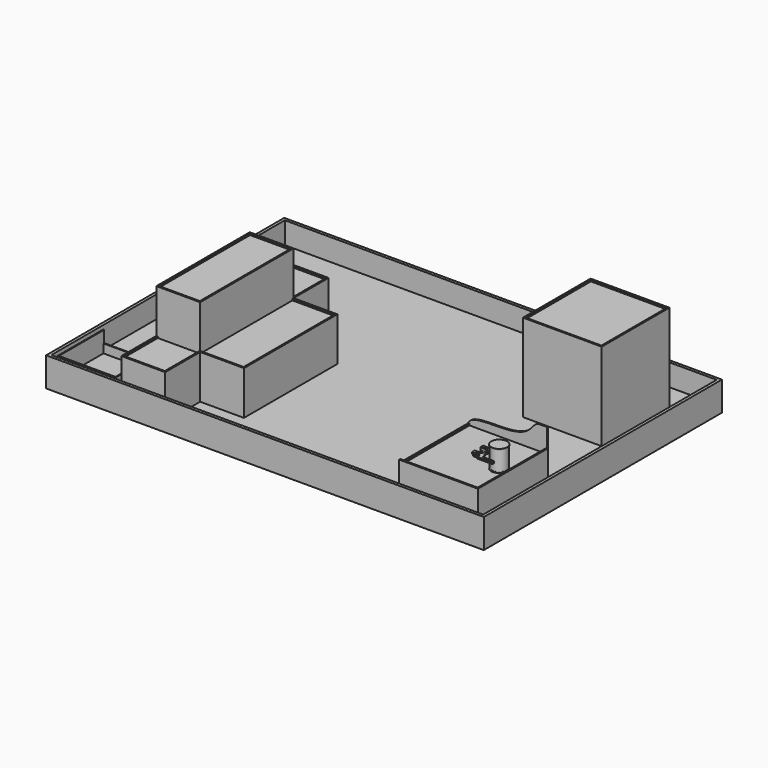
from build123d import *

# Parameters (mm, degrees)
F0_R      = 27.2
F1_DEPTH  = 2.83
F2_R      = 26.4
F3_DEPTH  = 67.36
F4_R      = 27.2
F5_DEPTH  = 2.83
F9_W      = 270
F9_H      = 300
F10_DEPTH = 72
F12_DEPTH = 15
F14_DEPTH = 5
F15_W     = 5
F15_H     = 290
F16_DEPTH = 5
F17_W     = 1500
F17_H     = 1020
F18_DEPTH = 25
F19_W     = 270
F19_H     = 290
F20_DEPTH = 300
F21_W     = 260
F21_H     = 280
F22_DEPTH = 5
F23_W     = 1500
F23_H     = 1020
F23_W_2   = 1480
F23_H_2   = 1000
F24_DEPTH = 75
F26_DEPTH = 150
F27_W     = 150
F27_H     = 400
F28_DEPTH = 150
F29_W     = 140
F29_H     = 390
F30_DEPTH = 5
F31_W     = 140
F31_H     = 145
F31_W_2   = 145
F31_H_2   = 390
F32_DEPTH = 5
F33_R     = 3
F34_DEPTH = 4
F35_R     = 3.99999
F35_2_R   = 3.99999
F36_R     = 3
F37_DEPTH = 8
F38_R     = 3
F39_DEPTH = 8
F40_R     = 3
F40_R_2   = 2.5
F41_DEPTH = 3
F42_R     = 3
F42_R_2   = 2.5
F43_DEPTH = 3
F45_DEPTH = 270.001
F46_W     = 200
F46_H     = 200
F46_W_2   = 194
F46_H_2   = 191
F47_DEPTH = 30
F49_DEPTH = 40
F51_DEPTH = 6
F50_R     = 2.5
F53_DEPTH = 6


# Not quite as in the source:
# - a fillet or chamfer is up to 0.001 mm smaller than in the source, because OpenCascade refuses the exact size
# - a feature names something its author has since deleted; it is built from what else it names


with BuildPart() as f1:
    # F0 (on Top) → F1 (new body)
    with BuildSketch(Plane.XY):
        Circle(F0_R)
    extrude(amount=F1_DEPTH)

    # F2 (on face) → F3 (join)
    with BuildSketch(Plane.XY.offset(2.83)):
        Circle(F2_R)
    extrude(amount=F3_DEPTH)

    # F4 (on face) → F5 (join)
    with BuildSketch(Plane.XY.offset(70.19)):
        Circle(F4_R)
    extrude(amount=F5_DEPTH)


with BuildPart() as f10:
    # F9 (on Top) → F10 (new body)
    with BuildSketch(Plane.XY):
        with Locations((-87.8, 0)):
            Rectangle(F9_W, F9_H)
    extrude(amount=-F10_DEPTH)

    # F11 (on face) → F12 (join)
    with BuildSketch(Plane.XY):
        Polygon((-222.8, -145), (-222.8, -150), (47.2, -150), (47.2, 150), (42.2, 150), (42.2, -145), align=None)
    extrude(amount=F12_DEPTH)

    # F13 (on face) → F14 (join)
    with BuildSketch(Plane(origin=(0, 150, 0), x_dir=(-1, 0, 0), z_dir=(0, 1, 0))):
        with BuildLine():
            Line((-21.3134280931, 81.3575685024), (-47.2, 81.3575685024))
            Line((-47.2, 81.3575685024), (-47.2, -72))
            Line((-47.2, -72), (222.8, -72))
            Line((222.8, -72), (222.8, 0))
            add(Edge.make_bspline(
                [(-21.3134280931, 81.3575685024), (-6.3059147253, 81.3822787863), (12.9585432644, 38.1268753575), (103.6097013063, 23.6068887567), (223.0224295336, 30.7718731823), (222.8, 0)],
                knots=[0, 0, 0, 0, 0.2487100673, 0.6151112321, 1, 1, 1, 1], degree=3))
        make_face()
    extrude(amount=-F14_DEPTH)

    # F15 (on face) → F16 (join)
    with BuildSketch(Plane.XY):
        with Locations((-220.3, 0)):
            Rectangle(F15_W, F15_H)
    extrude(amount=F16_DEPTH)

    # F17 (on face) → F18 (join)
    with BuildSketch(Plane(origin=(0, 0, -72), x_dir=(1, 0, 0), z_dir=(0, 0, -1))):
        with Locations((-602.8, -260)):
            Rectangle(F17_W, F17_H)
    extrude(amount=F18_DEPTH)

    # F19 (on face) → F20 (join)
    with BuildSketch(Plane.XY.offset(-72)):
        with Locations((-87.8, 525)):
            Rectangle(F19_W, F19_H)
    extrude(amount=F20_DEPTH)

    # F21 (on face) → F22 (cut)
    with BuildSketch(Plane.XY.offset(228)):
        with Locations((-87.8, 525)):
            Rectangle(F21_W, F21_H)
    extrude(amount=-F22_DEPTH, mode=Mode.SUBTRACT)

    # F23 (on face) → F24 (join)
    with BuildSketch(Plane.XY.offset(-72)):
        with Locations((-602.8, 260)):
            Rectangle(F23_W, F23_H)
        with Locations((-602.8, 260)):
            Rectangle(F23_W_2, F23_H_2, mode=Mode.SUBTRACT)
    extrude(amount=F24_DEPTH)

    # F25 (on face) → F26 (join)
    with BuildSketch(Plane.XY.offset(-72)):
        Polygon((-952.8, 460), (-1102.8, 460), (-1102.8, -240), (-952.8, -240), (-952.8, -90), (-802.8, -90), (-802.8, 310), (-952.8, 310), align=None)
    extrude(amount=F26_DEPTH)

    # F27 (on face) → F28 (join)
    with BuildSketch(Plane.XY.offset(78)):
        with Locations((-1027.8, 110)):
            Rectangle(F27_W, F27_H)
    extrude(amount=F28_DEPTH)

    # F29 (on face) → F30 (cut)
    with BuildSketch(Plane.XY.offset(228)):
        with Locations((-1027.8, 110)):
            Rectangle(F29_W, F29_H)
    extrude(amount=-F30_DEPTH, mode=Mode.SUBTRACT)

    # F31 (on face) → F32 (cut)
    with BuildSketch(Plane.XY.offset(78)):
        with Locations((-1027.8, 382.5)):
            Rectangle(F31_W, F31_H)
        with Locations((-880.3, 110)):
            Rectangle(F31_W_2, F31_H_2)
        with Locations((-1027.8, -162.5)):
            Rectangle(F31_W, F31_H)
    extrude(amount=-F32_DEPTH, mode=Mode.SUBTRACT)

    # F46 (on face) → F47 (join)
    with BuildSketch(Plane.XY.offset(-72)):
        with Locations((-1232.8, -130)):
            Rectangle(F46_W, F46_H)
        with Locations((-1232.8, -128.5)):
            Rectangle(F46_W_2, F46_H_2, mode=Mode.SUBTRACT)
    extrude(amount=F47_DEPTH)

    # F48 (on face) → F49 (join)
    with BuildSketch(Plane.XY.offset(-42)):
        Polygon((-1329.8, -30), (-1332.8, -30), (-1332.8, -230), (-1329.8, -230), (-1135.8, -230), (-1132.8, -230), (-1132.8, -30), (-1135.8, -30), (-1135.8, -224), (-1329.8, -224), align=None)
    extrude(amount=F49_DEPTH)


with BuildPart() as f34:
    # F33 (on offset) → F34 (new body, symmetric)
    with BuildSketch(Plane.XY.offset(25)):
        with BuildLine():
            Line((-55, -12), (-74.5, -12))
            Line((-74.5, -12), (-74.5, -13))
            Line((-74.5, -13), (-65.6457513111, -13))
            ThreePointArc((-65.6457513111, -13), (-67, -16), (-65.6457513111, -19))
            Line((-65.6457513111, -19), (-74.5, -19))
            Line((-74.5, -19), (-74.5, -20))
            Line((-74.5, -20), (-55, -20))
            ThreePointArc((-55, -20), (-51, -16), (-55, -12))
        make_face()
        with Locations((-63, -16)):
            Circle(F33_R, mode=Mode.SUBTRACT)
        with Locations((-55, -16)):
            Circle(F33_R, mode=Mode.SUBTRACT)
    extrude(amount=F34_DEPTH, both=True)

    # F35 (radius 4 in the source; OpenCascade refuses exactly that, so slightly less here)
    f35_edges = [f34.edges().sort_by_distance(p)[0] for p in [
        (-74.5, -19.5, 29),
        (-74.5, -12.5, 29),
        (-74.5, -19.5, 21),
        (-74.5, -12.5, 21),
    ]]
    fillet(f35_edges, radius=F35_R)

    # F36 (on face) → F37 (join, through all)
    with BuildSketch(Plane.XZ.offset(20)):
        with Locations((-70.5, 25)):
            Circle(F36_R)
    extrude(amount=-F37_DEPTH)

    # F42 (on offset) → F43 (join, symmetric)
    with BuildSketch(Plane.XY.offset(25)):
        with Locations((-63, -16)):
            Circle(F42_R)
        with Locations((-63, -16)):
            Circle(F42_R_2, mode=Mode.SUBTRACT)
        with Locations((-55, -16)):
            Circle(F42_R)
        with Locations((-55, -16)):
            Circle(F42_R_2, mode=Mode.SUBTRACT)
    extrude(amount=F43_DEPTH, both=True)


with BuildPart() as f34b:
    # F33 (on offset) → F34, piece 2 (new body, symmetric)
    with BuildSketch(Plane.XY.offset(25)):
        with BuildLine():
            Line((-74.5, 13), (-74.5, 12))
            Line((-74.5, 12), (-55, 12))
            ThreePointArc((-55, 12), (-51, 16), (-55, 20))
            Line((-55, 20), (-74.5, 20))
            Line((-74.5, 20), (-74.5, 19))
            Line((-74.5, 19), (-65.6457513111, 19))
            ThreePointArc((-65.6457513111, 19), (-67, 16), (-65.6457513111, 13))
            Line((-65.6457513111, 13), (-74.5, 13))
        make_face()
        with Locations((-63, 16)):
            Circle(F33_R, mode=Mode.SUBTRACT)
        with Locations((-55, 16)):
            Circle(F33_R, mode=Mode.SUBTRACT)
    extrude(amount=F34_DEPTH, both=True)

    # F35#2 (radius 4 in the source; OpenCascade refuses exactly that, so slightly less here)
    f35_2_edges = [f34b.edges().sort_by_distance(p)[0] for p in [
        (-74.5, 12.5, 29),
        (-74.5, 19.5, 29),
        (-74.5, 19.5, 21),
        (-74.5, 12.5, 21),
    ]]
    fillet(f35_2_edges, radius=F35_2_R)

    # F38 (on face) → F39 (join, through all)
    with BuildSketch(Plane(origin=(0, 20, 0), x_dir=(-1, 0, 0), z_dir=(0, 1, 0))):
        with Locations((70.5, 25)):
            Circle(F38_R)
    extrude(amount=-F39_DEPTH)

    # F40 (on offset) → F41 (join, symmetric)
    with BuildSketch(Plane.XY.offset(25)):
        with Locations((-55, 16)):
            Circle(F40_R)
        with Locations((-55, 16)):
            Circle(F40_R_2, mode=Mode.SUBTRACT)
        with Locations((-63, 16)):
            Circle(F40_R)
        with Locations((-63, 16)):
            Circle(F40_R_2, mode=Mode.SUBTRACT)
    extrude(amount=F41_DEPTH, both=True)


with BuildPart() as f45_tool:
    # F44 (on face) → F45 (new body, through all)
    with BuildSketch(Plane(origin=(0, 20, 0), x_dir=(-1, 0, 0), z_dir=(0, 1, 0))):
        with BuildLine():
            Line((71.5, 26), (71.5, 27.2912878475))
            ThreePointArc((71.5, 27.2912878475), (70.5, 27.5), (69.5, 27.2912878475))
            Line((69.5, 27.2912878475), (69.5, 26))
            Line((69.5, 26), (68.2087121525, 26))
            ThreePointArc((68.2087121525, 26), (68, 25), (68.2087121525, 24))
            Line((68.2087121525, 24), (69.5, 24))
            Line((69.5, 24), (69.5, 22.7087121525))
            ThreePointArc((69.5, 22.7087121525), (70.5, 22.5), (71.5, 22.7087121525))
            Line((71.5, 22.7087121525), (71.5, 24))
            Line((71.5, 24), (72.7912878475, 24))
            ThreePointArc((72.7912878475, 24), (73, 25), (72.7912878475, 26))
            Line((72.7912878475, 26), (71.5, 26))
        make_face()
    extrude(amount=-F45_DEPTH)


with BuildPart() as f34_1:
    add(f34.part)

    # F45: cut by f45_tool
    add(f45_tool.part, mode=Mode.SUBTRACT)


with BuildPart() as f34b_1:
    add(f34b.part)

    # F45: cut by f45_tool
    add(f45_tool.part, mode=Mode.SUBTRACT)


with BuildPart() as f51:
    # F50 (on face) → F51 (new body)
    with BuildSketch(Plane.XY.offset(29)):
        with BuildLine():
            ThreePointArc((-34.0286903083, 20.2639267135), (-34.1723386864, 20.1324758346), (-34.3150423771, 20))
            Line((-34.3150423771, 20), (-34.0286903083, 20))
            Line((-34.0286903083, 20), (-34.0286903083, 20.2639267135))
        make_face()
    extrude(amount=F51_DEPTH)


with BuildPart() as f51b:
    # F50 (on face) → F51, piece 2 (new body)
    with BuildSketch(Plane.XY.offset(29)):
        with BuildLine():
            Line((-34.3150423771, 20), (-74.2819495499, 20))
            Line((-74.2819495499, 20), (-74.2819495499, 12))
            Line((-74.2819495499, 12), (-48.7203188241, 12))
            Line((-48.7203188241, 12), (-48.7203188241, -12))
            Line((-48.7203188241, -12), (-74.2819495499, -12))
            Line((-74.2819495499, -12), (-74.2819495499, -20))
            Line((-74.2819495499, -20), (-34.0286903083, -20))
            ThreePointArc((-34.0286903083, -20), (-42.9374479461, -0.0627510607), (-34.3150423771, 20))
        make_face()
        with Locations((-63, -16)):
            Circle(F50_R, mode=Mode.SUBTRACT)
        with Locations((-55, -16)):
            Circle(F50_R, mode=Mode.SUBTRACT)
        with Locations((-63, 16)):
            Circle(F50_R, mode=Mode.SUBTRACT)
        with Locations((-55, 16)):
            Circle(F50_R, mode=Mode.SUBTRACT)
    extrude(amount=F51_DEPTH)

    # F52 (on face) → F53 (join)
    with BuildSketch(Plane.XY.offset(35)):
        Polygon((-74.2819495499, 20), (-34.3150423771, 20), (-34.3150423771, 27.871824801), (4.6629640274, 27.871824801), (4.6629640274, 35.8570814133), (-47.2162887454, 35.8570814133), (-47.2162887454, 23.757994175), (-74.2819495499, 23.757994175), align=None)
        Polygon((-47.2162887454, -24.0915641189), (-47.2162887454, -35.8570814133), (4.6629640274, -35.8570814133), (4.6629640274, -27.871824801), (-34.0286903083, -27.871824801), (-34.0286903083, -20), (-74.2819495499, -20), (-74.2819495499, -24.0915641189), align=None)
    extrude(amount=-F53_DEPTH)


solid = Compound([f1.part, f10.part, f34_1.part, f34b_1.part, f51.part, f51b.part])
